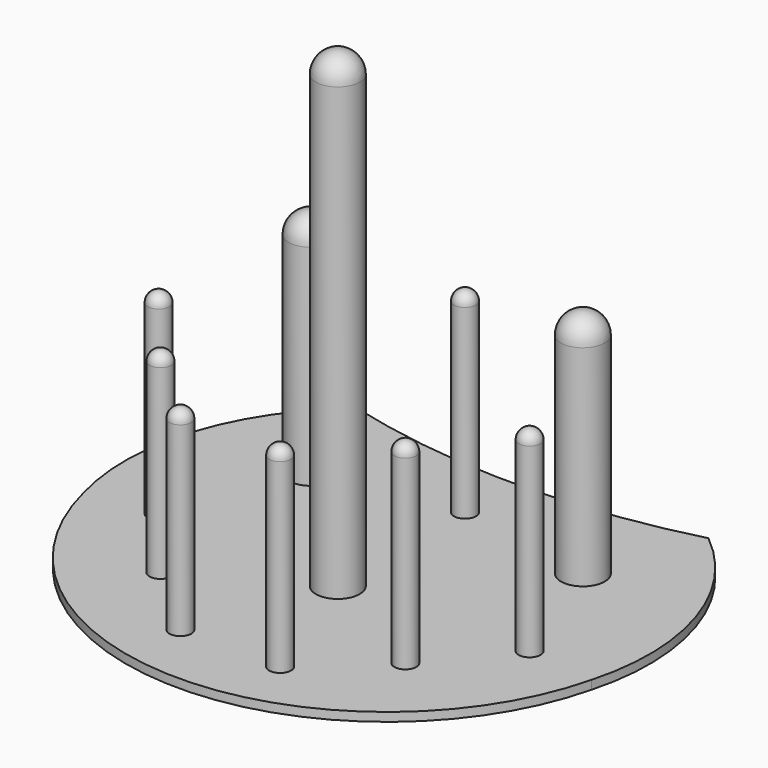
from build123d import *

# Parameters (mm, degrees)
F0_R     = 2.5
F0_R_2   = 20
F0_R_3   = 5
F1_DEPTH = 2
F2_DEPTH = 47
F3_DEPTH = 110
F4_DEPTH = 55
F5_R     = 2.5
F6_R     = 5


with BuildPart() as f1:
    # F0 (on Top) → F1 (new body)
    with BuildSketch(Plane.XY):
        with BuildLine():
            ThreePointArc((-40.0922639073, 55.7496552601), (-57.3483186907, 30.5416310101), (-58, 0))
            ThreePointArc((-58, 0), (0, -45.5817599767), (58, 0))
            ThreePointArc((58, 0), (57.3483186907, 30.5416310101), (40.0922639073, 55.7496552601))
            ThreePointArc((40.0922639073, 55.7496552601), (0, 50.5905433091), (-40.0922639073, 55.7496552601))
        make_face()
        with Locations((-11.3973486953, -30.7189605409)):
            Circle(F0_R, mode=Mode.SUBTRACT)
        with Locations((-42.3908012718, 1.806866884)):
            Circle(F0_R, mode=Mode.SUBTRACT)
        with Locations((-27.9805496199, -15.6816352416)):
            Circle(F0_R, mode=Mode.SUBTRACT)
        with Locations((11.3973486953, -30.7189605409)):
            Circle(F0_R, mode=Mode.SUBTRACT)
        with Locations((27.9805496199, -15.6816352416)):
            Circle(F0_R, mode=Mode.SUBTRACT)
        Circle(F0_R_2, mode=Mode.SUBTRACT)
        with Locations((42.3908012718, 1.806866884)):
            Circle(F0_R, mode=Mode.SUBTRACT)
        with Locations((-31.1126983722, 31.1126983722)):
            Circle(F0_R_2, mode=Mode.SUBTRACT)
        with Locations((-0.0906402458, 36.447709117)):
            Circle(F0_R, mode=Mode.SUBTRACT)
        with Locations((31.1126983722, 31.1126983722)):
            Circle(F0_R_2, mode=Mode.SUBTRACT)
        Circle(F0_R_2)
        Circle(F0_R_3, mode=Mode.SUBTRACT)
        with Locations((-31.1126983722, 31.1126983722)):
            Circle(F0_R_2)
        with Locations((-31.1126983722, 31.1126983722)):
            Circle(F0_R_3, mode=Mode.SUBTRACT)
        with Locations((31.1126983722, 31.1126983722)):
            Circle(F0_R_2)
        with Locations((31.1126983722, 31.1126983722)):
            Circle(F0_R_3, mode=Mode.SUBTRACT)
    extrude(amount=F1_DEPTH)

    # F0 (on Top) → F2 (join)
    with BuildSketch(Plane.XY):
        with Locations((11.3973486953, -30.7189605409)):
            Circle(F0_R)
        with Locations((-11.3973486953, -30.7189605409)):
            Circle(F0_R)
        with Locations((-27.9805496199, -15.6816352416)):
            Circle(F0_R)
        with Locations((-42.3908012718, 1.806866884)):
            Circle(F0_R)
        with Locations((27.9805496199, -15.6816352416)):
            Circle(F0_R)
        with Locations((42.3908012718, 1.806866884)):
            Circle(F0_R)
        with Locations((-0.0906402458, 36.447709117)):
            Circle(F0_R)
    extrude(amount=F2_DEPTH)

    # F0 (on Top) → F3 (join)
    with BuildSketch(Plane.XY):
        Circle(F0_R_3)
    extrude(amount=F3_DEPTH)

    # F0 (on Top) → F4 (join)
    with BuildSketch(Plane.XY):
        with Locations((31.1126983722, 31.1126983722)):
            Circle(F0_R_3)
        with Locations((-31.1126983722, 31.1126983722)):
            Circle(F0_R_3)
    extrude(amount=F4_DEPTH)

    # F5
    f5_edges = [f1.edges().sort_by_distance(p)[0] for p in [
        (-30.48055, -15.681635, 47),
        (-44.890801, 1.806867, 47),
        (-13.897349, -30.718961, 47),
        (8.897349, -30.718961, 47),
        (25.48055, -15.681635, 47),
        (39.890801, 1.806867, 47),
        (-2.59064, 36.447709, 47),
    ]]
    fillet(f5_edges, radius=F5_R)

    # F6
    f6_edges = [f1.edges().sort_by_distance(p)[0] for p in [
        (5, 0, 56),
        (26.112698, 31.112698, 55),
        (-36.112698, 31.112698, 55),
        (-5, 0, 110),
    ]]
    fillet(f6_edges, radius=F6_R)

    # F7 (on Front) → F8 (revolve, cut)
    with BuildSketch(Plane.XZ):
        with BuildLine():
            Line((-1.8863899168, 95.4484194517), (-1.8863899168, 12.7471061423))
            ThreePointArc((-1.8863899168, 12.7471061423), (-1.4088517979, 8.4923255002), (0, 4.4492650777))
            Line((0, 4.4492650777), (0, 103.6416590214))
            ThreePointArc((0, 103.6416590214), (-1.4087030362, 99.6522165913), (-1.8863899168, 95.4484194517))
        make_face()
    revolve(axis=Axis((0, 0, 54.0454620495), (0, 0, 1)), mode=Mode.SUBTRACT)

    # F10 (on offset) → F11 (revolve, cut)
    with BuildSketch(Plane.XZ.offset(-31.113)):
        with BuildLine():
            ThreePointArc((28.3645223826, 18.5954442493), (28.6747148829, 11.4377864347), (31.1126983722, 4.7009829432))
            Line((31.1126983722, 4.7009829432), (31.1126983722, 43.899834156))
            ThreePointArc((31.1126983722, 43.899834156), (29.0593154607, 37.6495133595), (28.3645223826, 31.1073306948))
            Line((28.3645223826, 31.1073306948), (28.3645223826, 18.5954442493))
        make_face()
    revolve(axis=Axis((31.1126983722, 31.113, 24.3004085496), (0, 0, 1)), mode=Mode.SUBTRACT)

    # F10 (on offset) → F12 (revolve, cut)
    with BuildSketch(Plane.XZ.offset(-31.113)):
        with BuildLine():
            ThreePointArc((-33.8608743618, 18.5954442493), (-33.5506818615, 11.4377864347), (-31.1126983722, 4.7009829432))
            Line((-31.1126983722, 4.7009829432), (-31.1126983722, 43.899834156))
            ThreePointArc((-31.1126983722, 43.899834156), (-33.1660812837, 37.6495133595), (-33.8608743618, 31.1073306948))
            Line((-33.8608743618, 31.1073306948), (-33.8608743618, 18.5954442493))
        make_face()
    revolve(axis=Axis((-31.1126983722, 31.113, 24.3004085496), (0, 0, 1)), mode=Mode.SUBTRACT)


solid = f1.part
